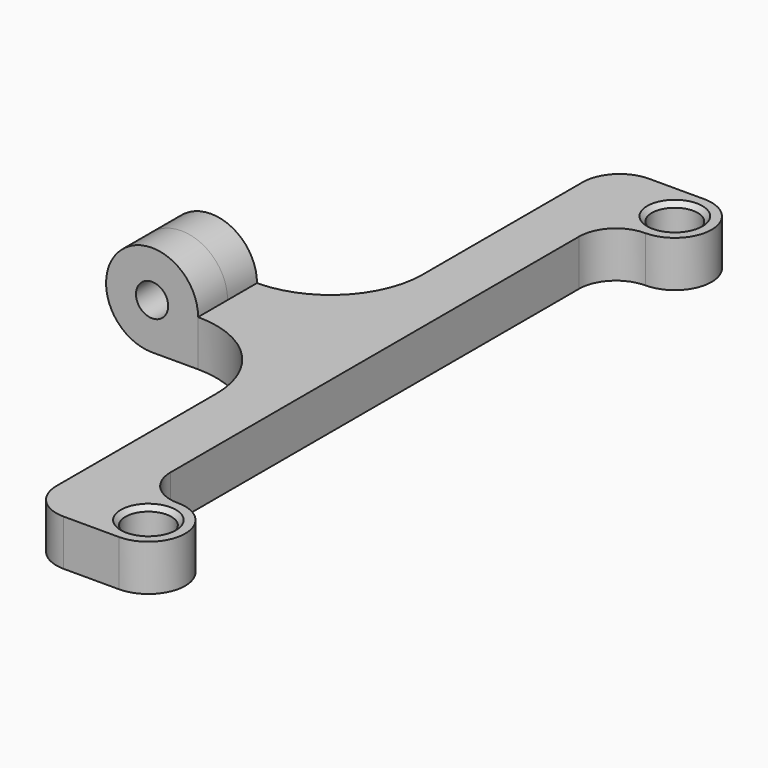
from build123d import *

# Parameters (mm, degrees)
F0_R          = 2.5
F1_DEPTH      = 5
F2_R          = 5
F3_DEPTH      = 4
F3_DEPTH_BACK = 4
F4_R          = 1.75
F5_DEPTH      = 39.751
F5_DEPTH_BACK = 39.751
F6_SIZE       = 0.5


# Not quite as in the source:
# - after a boolean that leaves OpenCascade's solid faulty, fix() repairs it


with BuildPart() as f1:
    # F0 (on Top) → F1 (new body)
    with BuildSketch(Plane.XY):
        with BuildLine():
            Line((-16, 4), (-26, 4))
            Line((-26, 4), (-26, 0))
            Line((-26, 0), (-26, -4))
            Line((-26, -4), (-16, -4))
            ThreePointArc((-16, -4), (-8.9289321881, -6.9289321881), (-6, -14))
            Line((-6, -14), (-6, -35.75))
            ThreePointArc((-6, -35.75), (-4.8284271247, -38.5784271247), (-2, -39.75))
            Line((-2, -39.75), (4, -39.75))
            ThreePointArc((4, -39.75), (8, -35.75), (4, -31.75))
            ThreePointArc((4, -31.75), (1.1715728753, -30.5784271247), (0, -27.75))
            Line((0, -27.75), (0, 0))
            Line((0, 0), (0, 27.75))
            ThreePointArc((0, 27.75), (1.1715728753, 30.5784271247), (4, 31.75))
            ThreePointArc((4, 31.75), (8, 35.75), (4, 39.75))
            Line((4, 39.75), (-2, 39.75))
            ThreePointArc((-2, 39.75), (-4.8284271247, 38.5784271247), (-6, 35.75))
            Line((-6, 35.75), (-6, 14))
            ThreePointArc((-6, 14), (-8.9289321881, 6.9289321881), (-16, 4))
        make_face()
        with Locations((4, -35.75)):
            Circle(F0_R, mode=Mode.SUBTRACT)
        with Locations((4, 35.75)):
            Circle(F0_R, mode=Mode.SUBTRACT)
    extrude(amount=F1_DEPTH)

    # F2 (on Front) → F3 (join, two sides)
    with BuildSketch(Plane.XZ) as f3_sk:
        with Locations((-21, 5)):
            Circle(F2_R)
    extrude(amount=F3_DEPTH)
    extrude(f3_sk.sketch, amount=-F3_DEPTH_BACK)

    # F4 (on Front) → F5 (cut, two sides)
    with BuildSketch(Plane.XZ) as f5_sk:
        with BuildLine():
            ThreePointArc((-21, 0), (-24.5355339059, 1.4644660941), (-26, 5))
            Line((-26, 5), (-26, 0))
            Line((-26, 0), (-21, 0))
        make_face()
        with Locations((-21, 5)):
            Circle(F4_R)
    extrude(amount=-F5_DEPTH, mode=Mode.SUBTRACT)
    extrude(f5_sk.sketch, amount=F5_DEPTH_BACK, mode=Mode.SUBTRACT)

    add(f1.part.fix(), mode=Mode.REPLACE)

    # F6
    f6_edges = [f1.edges().sort_by_distance(p)[0] for p in [
        (1.5, 35.75, 5),
        (1.5, -35.75, 5),
    ]]
    chamfer(f6_edges, length=F6_SIZE)


solid = f1.part
